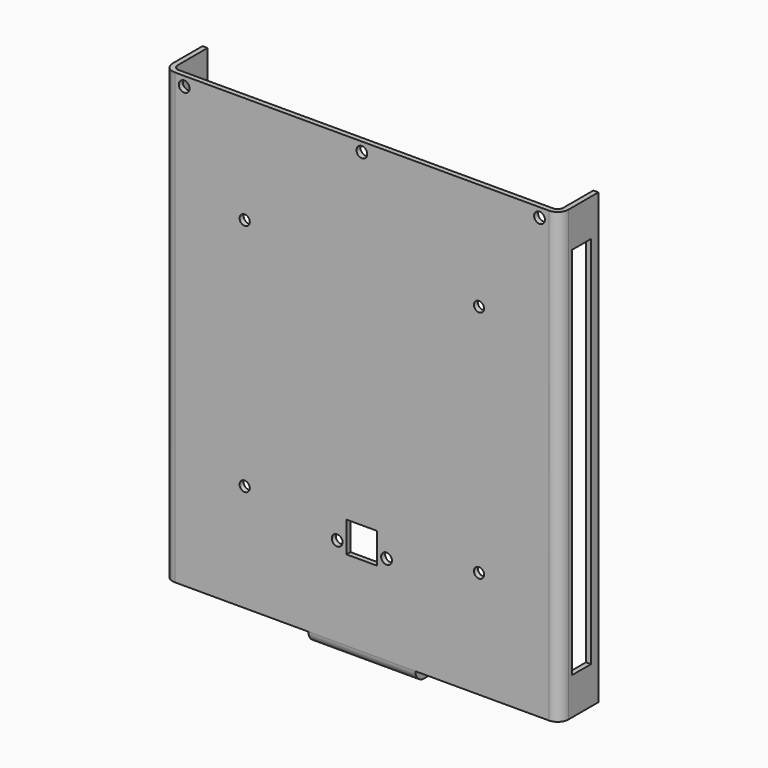
from build123d import *

# Parameters (mm, degrees)
F1_DEPTH  = 152.4
F2_W      = 7.9375
F2_H      = 127.0931567346
F3_DEPTH  = 134.38632
F4_W      = 36.322
F4_H      = 1.70942
F5_DEPTH  = 3.69316
F6_W      = 36.322
F6_H      = 1.70942
F7_DEPTH  = 33.4645
F8_R      = 3.69316
F9_R      = 1.98374
F10_R     = 5.969
F10_R_2   = 1.5
F11_DEPTH = 3.69316
F12_R     = 18.16099
F13_R     = 1.8288
F14_DEPTH = 1.70942
F15_R     = 1.7272
F16_DEPTH = 1.70942
F17_W     = 10.40892
F17_H     = 10.40892
F17_R     = 1.8288
F18_DEPTH = 1.70942


# Not quite as in the source:
# - a fillet or chamfer is up to 0.001 mm smaller than in the source, because OpenCascade refuses the exact size


with BuildPart() as f1:
    # F0 (on Top) → F1 (new body)
    with BuildSketch(Plane.XY):
        Polygon((0, 14.68374), (0, 0), (-130.96748, 0), (-130.96748, 14.68374), (-132.6769, 14.68374), (-132.6769, -1.70942), (1.70942, -1.70942), (1.70942, 14.68374), align=None)
    extrude(amount=F1_DEPTH)

    # F2 (on face) → F3 (cut, through all)
    with BuildSketch(Plane.YZ.offset(1.70942)):
        with Locations((7.53999, 76.2)):
            Rectangle(F2_W, F2_H)
    extrude(amount=-F3_DEPTH, mode=Mode.SUBTRACT)

    # F4 (on face) → F5 (join)
    with BuildSketch(Plane(origin=(0, 0, 0), x_dir=(1, 0, 0), z_dir=(0, 0, -1))):
        with Locations((-65.48374, 0.85471)):
            Rectangle(F4_W, F4_H)
    extrude(amount=F5_DEPTH)

    # F6 (on face) → F7 (join)
    with BuildSketch(Plane(origin=(0, 0, 0), x_dir=(-1, 0, 0), z_dir=(0, 1, 0))):
        with Locations((65.48374, -2.83845)):
            Rectangle(F6_W, F6_H)
    extrude(amount=F7_DEPTH)

    # F8
    f8_edges = [f1.edges().sort_by_distance(p)[0] for p in [
        (1.70942, -1.70942, 76.2),
        (-132.6769, -1.70942, 76.2),
        (-65.48374, -1.70942, -3.69316),
    ]]
    fillet(f8_edges, radius=F8_R)

    # F9
    f9_edges = [f1.edges().sort_by_distance(p)[0] for p in [
        (0, 0, 76.2),
        (-130.96748, 0, 76.2),
        (-65.48374, 0, -1.98374),
    ]]
    fillet(f9_edges, radius=F9_R)

    # F10 (on face) → F11 (cut, through all)
    with BuildSketch(Plane(origin=(0, 0, -3.69316), x_dir=(1, 0, 0), z_dir=(0, 0, -1))):
        with Locations((-65.48374, -7.9375)):
            Circle(F10_R)
        with Locations((-49.9897398917, -15.3035)):
            Circle(F10_R_2)
        with Locations((-80.9777401083, -15.3035)):
            Circle(F10_R_2)
        with Locations((-73.2307400541, -28.7216977)):
            Circle(F10_R_2)
        with Locations((-57.7367399459, -28.7216977)):
            Circle(F10_R_2)
    extrude(amount=-F11_DEPTH, mode=Mode.SUBTRACT)

    # F12 (radius 18.161 in the source; OpenCascade refuses exactly that, so slightly less here)
    f12_edges = [f1.edges().sort_by_distance(p)[0] for p in [
        (-47.32274, 33.4645, -2.83845),
        (-83.64474, 33.4645, -2.83845),
    ]]
    fillet(f12_edges, radius=F12_R)

    # F13 (on face) → F14 (cut, through all)
    with BuildSketch(Plane.XZ.offset(1.70942)):
        with Locations((-65.48374, 149.225)):
            Circle(F13_R)
        with Locations((-5.15874, 149.225)):
            Circle(F13_R)
        with Locations((-125.80874, 149.225)):
            Circle(F13_R)
    extrude(amount=-F14_DEPTH, mode=Mode.SUBTRACT)

    # F15 (on face) → F16 (cut, through all)
    with BuildSketch(Plane.XZ.offset(1.70942)):
        with Locations((-105.2585017, 115.9747617)):
            Circle(F15_R)
        with Locations((-25.7089783, 115.9747617)):
            Circle(F15_R)
        with Locations((-25.7089783, 36.4252383)):
            Circle(F15_R)
        with Locations((-105.2585017, 36.4252383)):
            Circle(F15_R)
    extrude(amount=-F16_DEPTH, mode=Mode.SUBTRACT)

    # F17 (on face) → F18 (cut, through all)
    with BuildSketch(Plane(origin=(0, 0, 0), x_dir=(-1, 0, 0), z_dir=(0, 1, 0))):
        with Locations((65.48374, 32.4986058015)):
            Rectangle(F17_W, F17_H)
        with Locations((73.8632, 30.4691458015)):
            Circle(F17_R)
        with Locations((57.10428, 30.4691458015)):
            Circle(F17_R)
    extrude(amount=-F18_DEPTH, mode=Mode.SUBTRACT)


solid = f1.part
